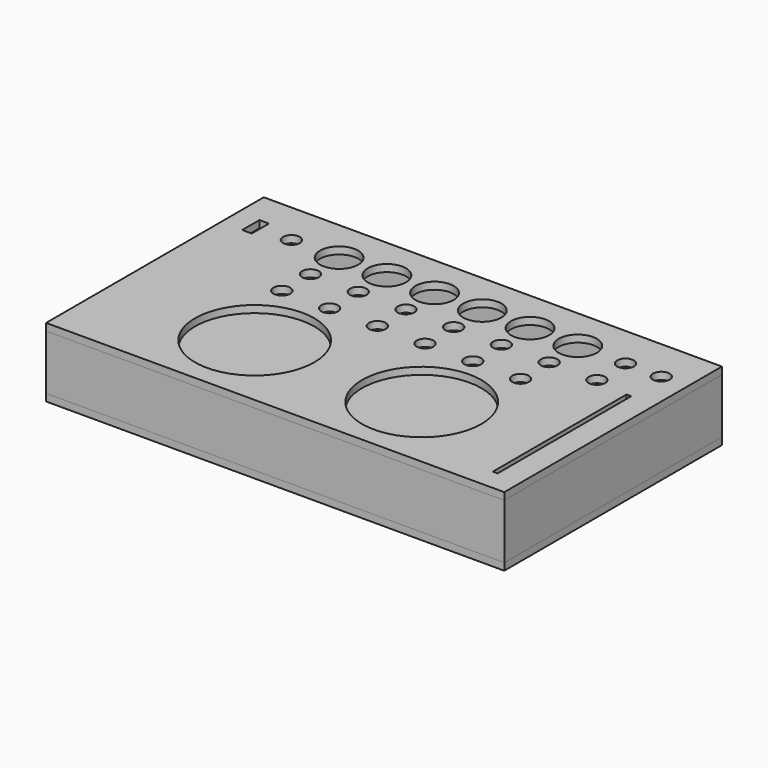
from build123d import *

# Parameters (mm, degrees)
F1_W     = 192
F1_H     = 114
F1_W_2   = 186
F1_H_2   = 108
F2_DEPTH = 23
F1_R     = 25
F1_W_3   = 10
F1_H_3   = 75
F1_R_2   = 3.5
F1_W_4   = 4
F1_H_4   = 9
F1_R_3   = 8
F1_W_5   = 17
F1_H_5   = 20
F1_W_6   = 2
F1_H_6   = 70
F3_DEPTH = 3
F4_W     = 192
F4_H     = 114
F4_W_2   = 186
F4_H_2   = 108
F5_DEPTH = 3


# Not quite as in the source:
# - a feature names something its author has since deleted; it is built from what else it names


with BuildPart() as f2:
    # F1 (on Top) → F2 (new body)
    with BuildSketch(Plane.XY):
        with Locations((-5.0508876443, 0.7905893784)):
            Rectangle(F1_W, F1_H)
        with Locations((-5.0508876443, 0.7905893784)):
            Rectangle(F1_W_2, F1_H_2, mode=Mode.SUBTRACT)
    extrude(amount=-F2_DEPTH)


with BuildPart() as f3:
    # F1 (on Top) → F3 (new body)
    with BuildSketch(Plane.XY):
        with Locations((-5.0508876443, 0.7905893784)):
            Rectangle(F1_W, F1_H)
        with Locations((-5.0508876443, 0.7905893784)):
            Rectangle(F1_W_2, F1_H_2, mode=Mode.SUBTRACT)
        with Locations((-5.0508876443, 0.7905893784)):
            Rectangle(F1_W_2, F1_H_2)
        with Locations((-40.0508876443, -23.2094106216)):
            Circle(F1_R, mode=Mode.SUBTRACT)
        with Locations((29.9491123557, -23.2094106216)):
            Circle(F1_R, mode=Mode.SUBTRACT)
        with Locations((79.9491123557, -12.2163163405)):
            Rectangle(F1_W_3, F1_H_3, mode=Mode.SUBTRACT)
        with Locations((-55.0508876443, 9.7905893784)):
            Circle(F1_R_2, mode=Mode.SUBTRACT)
        with Locations((-55.0508876443, 24.7905893784)):
            Circle(F1_R_2, mode=Mode.SUBTRACT)
        with Locations((-35.0508876443, 9.7905893784)):
            Circle(F1_R_2, mode=Mode.SUBTRACT)
        with Locations((-15.0508876443, 9.7905893784)):
            Circle(F1_R_2, mode=Mode.SUBTRACT)
        with Locations((-35.0508876443, 24.7905893784)):
            Circle(F1_R_2, mode=Mode.SUBTRACT)
        with Locations((-15.0508876443, 24.7905893784)):
            Circle(F1_R_2, mode=Mode.SUBTRACT)
        with Locations((-90.0508876443, 39.7905893784)):
            Rectangle(F1_W_4, F1_H_4, mode=Mode.SUBTRACT)
        with Locations((-75.0508876443, 39.7905893784)):
            Circle(F1_R_2, mode=Mode.SUBTRACT)
        with Locations((-55.0508876443, 39.7905893784)):
            Circle(F1_R_3, mode=Mode.SUBTRACT)
        with Locations((-35.0508876443, 39.7905893784)):
            Circle(F1_R_3, mode=Mode.SUBTRACT)
        with Locations((-15.0508876443, 39.7905893784)):
            Circle(F1_R_3, mode=Mode.SUBTRACT)
        with Locations((4.9491123557, 9.7905893784)):
            Circle(F1_R_2, mode=Mode.SUBTRACT)
        with Locations((24.9491123557, 9.7905893784)):
            Circle(F1_R_2, mode=Mode.SUBTRACT)
        with Locations((4.9491123557, 24.7905893784)):
            Circle(F1_R_2, mode=Mode.SUBTRACT)
        with Locations((24.9491123557, 24.7905893784)):
            Circle(F1_R_2, mode=Mode.SUBTRACT)
        with Locations((64.9491123557, 3.2005797455)):
            Rectangle(F1_W_5, F1_H_5, mode=Mode.SUBTRACT)
        with Locations((44.9491123557, 9.7905893784)):
            Circle(F1_R_2, mode=Mode.SUBTRACT)
        with Locations((44.9491123557, 24.7905893784)):
            Circle(F1_R_2, mode=Mode.SUBTRACT)
        with Locations((64.9491123557, 24.7905893784)):
            Circle(F1_R_2, mode=Mode.SUBTRACT)
        with Locations((4.9491123557, 39.7905893784)):
            Circle(F1_R_3, mode=Mode.SUBTRACT)
        with Locations((24.9491123557, 39.7905893784)):
            Circle(F1_R_3, mode=Mode.SUBTRACT)
        with Locations((44.9491123557, 39.7905893784)):
            Circle(F1_R_3, mode=Mode.SUBTRACT)
        with Locations((64.9491123557, 39.7905893784)):
            Circle(F1_R_2, mode=Mode.SUBTRACT)
        with Locations((79.9491123557, 39.7905893784)):
            Circle(F1_R_2, mode=Mode.SUBTRACT)
        with Locations((64.9491123557, 3.2005797455)):
            Rectangle(F1_W_5, F1_H_5)
        with Locations((79.9491123557, -12.2163163405)):
            Rectangle(F1_W_3, F1_H_3)
        with Locations((79.9491123557, -12.2163163405)):
            Rectangle(F1_W_6, F1_H_6, mode=Mode.SUBTRACT)
    extrude(amount=F3_DEPTH)


with BuildPart() as f5:
    # F4 (on face) → F5 (new body)
    with BuildSketch(Plane(origin=(0, 0, -23), x_dir=(1, 0, 0), z_dir=(0, 0, -1))):
        with Locations((-5.0508876443, -0.7905893784)):
            Rectangle(F4_W, F4_H)
        with Locations((-5.0508876443, -0.7905893784)):
            Rectangle(F4_W_2, F4_H_2)
    extrude(amount=F5_DEPTH)


solid = Compound([f2.part, f3.part, f5.part])
